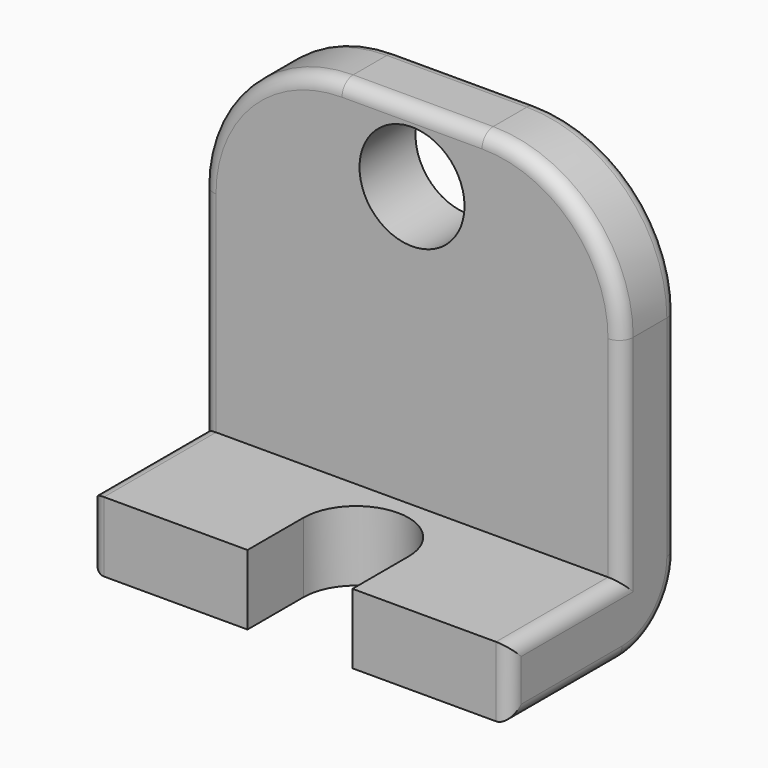
from build123d import *

# Parameters (mm, degrees)
F1_DEPTH      = 76.2
F1_DEPTH_BACK = 76.2
F2_R          = 19.05
F3_DEPTH      = 25.401
F5_DEPTH      = 25.401
F6_R          = 50.8
F7_R          = 5.08
F8_T1_DEPTH   = 152.4
F8_T4_ANGLE   = 90
F8_T6_ANGLE   = 90


# Not quite as in the source:
# - a fillet or chamfer that OpenCascade refuses, or shapes differently, is made with other operations: its cross-section is extruded or revolved along the edge and cut away or added


with BuildPart() as f1:
    # F0 (on Right) → F1 (new body, two sides)
    with BuildSketch(Plane.YZ) as f1_sk:
        Polygon((-76.2, 0), (0, 0), (0, 152.4), (-25.4, 152.4), (-25.4, 25.4), (-76.2, 25.4), align=None)
    extrude(amount=F1_DEPTH)
    extrude(f1_sk.sketch, amount=-F1_DEPTH_BACK)

    # F2 (on face) → F3 (cut, through all)
    with BuildSketch(Plane.XZ.offset(25.4)):
        with Locations((0, 127)):
            Circle(F2_R)
    extrude(amount=-F3_DEPTH, mode=Mode.SUBTRACT)

    # F4 (on face) → F5 (cut, through all)
    with BuildSketch(Plane.XY.offset(25.4)):
        with BuildLine():
            Line((19.05, -76.2), (19.05, -50.8))
            ThreePointArc((19.05, -50.8), (0, -69.85), (-19.05, -50.8))
            Line((-19.05, -50.8), (-19.05, -76.2))
            Line((-19.05, -76.2), (19.05, -76.2))
        make_face()
        with BuildLine():
            ThreePointArc((-19.05, -50.8), (0, -69.85), (19.05, -50.8))
            ThreePointArc((19.05, -50.8), (0, -31.75), (-19.05, -50.8))
        make_face()
    extrude(amount=-F5_DEPTH, mode=Mode.SUBTRACT)

    # F6
    f6_edges = [f1.edges().sort_by_distance(p)[0] for p in [
        (76.2, -12.7, 152.4),
        (-76.2, -12.7, 152.4),
    ]]
    fillet(f6_edges, radius=F6_R)

    # F7
    f7_edges = [f1.edges().sort_by_distance(p)[0] for p in [
        (61.321024, -25.4, 137.521024),
        (61.321024, 0, 137.521024),
        (76.2, -50.8, 25.4),
        (76.2, 0, 50.8),
        (76.2, -12.7, 101.6),
        (76.2, -38.1, 0),
        (76.2, -25.4, 63.5),
        (76.2, -76.2, 12.7),
        (-76.2, -50.8, 25.4),
        (-76.2, 0, 50.8),
        (-76.2, -12.7, 101.6),
        (-76.2, -38.1, 0),
        (-76.2, -25.4, 63.5),
        (-76.2, -76.2, 12.7),
    ]]
    fillet(f7_edges, radius=F7_R)

    # F8: fillet of radius 25.4 on 1 edges, made by hand

    # F8_s2 → F8_t1 (cut)
    with BuildSketch(Plane.YZ.offset(-76.2)):
        with BuildLine():
            ThreePointArc((0, 25.4), (-7.4394877579, 7.4394877579), (-25.4, 0))
            Line((-25.4, 0), (0, 0))
            Line((0, 0), (0, 25.4))
        make_face()
    extrude(amount=F8_T1_DEPTH, mode=Mode.SUBTRACT)

    # F8_s3 → F8_t4 (revolve, cut)
    with BuildSketch(Plane.XY.offset(25.4)):
        with BuildLine():
            ThreePointArc((-76.2, -5.08), (-74.7121024484, -1.4878975516), (-71.12, 0))
            Line((-71.12, 0), (-76.2, 0))
            Line((-76.2, 0), (-76.2, -5.08))
        make_face()
    revolve(axis=Axis((-76.2, -25.4, 25.4), (-1, 0, 0)), revolution_arc=F8_T4_ANGLE, mode=Mode.SUBTRACT)

    # F8_s5 → F8_t6 (revolve, cut)
    with BuildSketch(Plane.XZ.offset(25.4)):
        with BuildLine():
            ThreePointArc((76.2, 5.08), (74.7121024484, 1.4878975516), (71.12, 0))
            Line((71.12, 0), (76.2, 0))
            Line((76.2, 0), (76.2, 5.08))
        make_face()
    revolve(axis=Axis((76.2, -25.4, 25.4), (1, 0, 0)), revolution_arc=F8_T6_ANGLE, mode=Mode.SUBTRACT)


solid = f1.part
